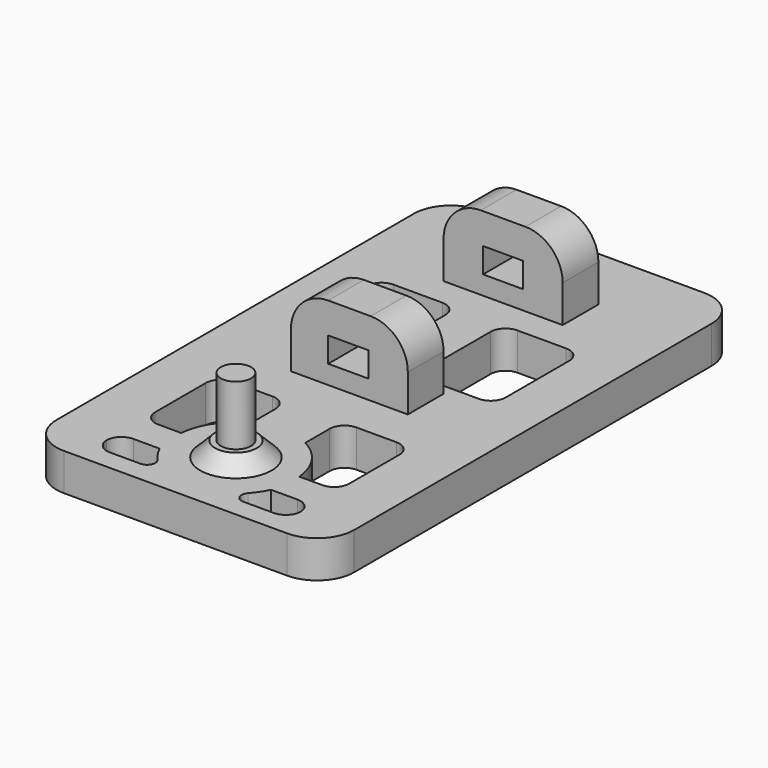
from build123d import *

# Parameters (mm, degrees)
F1_DEPTH     = 12.7
F3_DEPTH     = 25.4
F4_R         = 12.7
F5_R         = 12.7
F6_R         = 12.7
F8_DEPTH     = 104.141
F9_W         = 26.8278098665
F9_H         = 37.2433126904
F10_DEPTH    = 12.701
F11_R        = 5.08
F12_R        = 12.1917967362
F12_R_2      = 5.1797647995
F13_DEPTH    = 5.08
F14_DEPTH    = 25.4
F15_SIZE     = 5.07999
F17_DEPTH    = 25.4
F18_R        = 5.08
F19_DEPTH    = 12.701
F21_DEPTH    = 12.701
F22_T1_DEPTH = 12.7
F23_R        = 2.794


# Not quite as in the source:
# - a fillet or chamfer that OpenCascade refuses, or shapes differently, is made with other operations: its cross-section is extruded or revolved along the edge and cut away or added
# - a fillet or chamfer is up to 0.001 mm smaller than in the source, because OpenCascade refuses the exact size
# - a feature names something its author has since deleted; it is built from what else it names


with BuildPart() as f1:
    # F0 (on Top) → F1 (new body)
    with BuildSketch(Plane.XY):
        Polygon((-50.8, 88.9), (-50.8, 0), (-50.8, -88.9), (0, -88.9), (50.8, -88.9), (50.8, 0), (50.8, 88.9), (0, 88.9), align=None)
    extrude(amount=F1_DEPTH)

    # F2 (on face) → F3 (join)
    with BuildSketch(Plane.XY.offset(12.7)):
        Polygon((20.32, 66.04), (0, 66.04), (-20.32, 66.04), (-20.32, 50.8), (0, 50.8), (20.32, 50.8), align=None)
        Polygon((0, 0), (-19.5459036618, 0), (-19.5459036618, -15.24), (0, -15.24), (20.32, -15.24), (20.32, 0), align=None)
    extrude(amount=F3_DEPTH)

    # F4
    f4_edges = [f1.edges().sort_by_distance(p)[0] for p in [
        (20.32, -7.62, 38.1),
        (-19.545904, -7.62, 38.1),
    ]]
    fillet(f4_edges, radius=F4_R)

    # F5
    f5_edges = [f1.edges().sort_by_distance(p)[0] for p in [
        (20.32, 58.42, 38.1),
        (-20.32, 58.42, 38.1),
    ]]
    fillet(f5_edges, radius=F5_R)

    # F6
    f6_edges = [f1.edges().sort_by_distance(p)[0] for p in [
        (50.8, 88.9, 6.35),
        (-50.8, 88.9, 6.35),
        (50.8, -88.9, 6.35),
        (-50.8, -88.9, 6.35),
    ]]
    fillet(f6_edges, radius=F6_R)

    # F7 (on face) → F8 (cut, through all)
    with BuildSketch(Plane.XZ.offset(15.24)):
        Polygon((6.8459036618, 27.6168659329), (0, 27.6168659329), (-6.8459036618, 27.6168659329), (-6.8459036618, 19.0950892866), (0, 19.0950892866), (6.8459036618, 19.0950892866), align=None)
    extrude(amount=-F8_DEPTH, mode=Mode.SUBTRACT)

    # F9 (on face) → F10 (cut, through all)
    with BuildSketch(Plane.XY.offset(12.7)):
        with Locations((-21.1466264445, 22.2513012122)):
            Rectangle(F9_W, F9_H)
        with Locations((21.1466264445, 22.2513012122)):
            Rectangle(F9_W, F9_H)
    extrude(amount=-F10_DEPTH, mode=Mode.SUBTRACT)

    # F11
    f11_edges = [f1.edges().sort_by_distance(p)[0] for p in [
        (-34.560531, 40.872958, 6.35),
        (-7.732722, 40.872958, 6.35),
        (-7.732722, 3.629645, 6.35),
        (-34.560531, 3.629645, 6.35),
        (34.560531, 3.629645, 6.35),
        (7.732722, 3.629645, 6.35),
        (7.732722, 40.872958, 6.35),
        (34.560531, 40.872958, 6.35),
    ]]
    fillet(f11_edges, radius=F11_R)

    # F12 (on face) → F13 (join)
    with BuildSketch(Plane.XY.offset(12.7)):
        with Locations((0, -63.150562346)):
            Circle(F12_R)
        with Locations((0, -63.150562346)):
            Circle(F12_R_2, mode=Mode.SUBTRACT)
    extrude(amount=F13_DEPTH)

    # F14 (add): a face of the model
    f14_faces = [f1.faces().sort_by_distance(p)[0] for p in [
        (0, -63.150562346, 12.7),
    ]]
    extrude(f14_faces, amount=F14_DEPTH)

    # F15 (size 5.08 in the source; OpenCascade refuses exactly that, so slightly less here)
    f15_edges = [f1.edges().sort_by_distance(p)[0] for p in [
        (-12.191797, -63.150562, 17.78),
    ]]
    chamfer(f15_edges, length=F15_SIZE)

    # F16 (on face) → F17 (cut)
    with BuildSketch(Plane.XY.offset(12.7)):
        with BuildLine():
            Line((-9.2206190628, -29.6420995146), (-33.0726338262, -29.6420995146))
            Line((-33.0726338262, -29.6420995146), (-33.0726338262, -61.3056821097))
            Line((-33.0726338262, -61.3056821097), (-20.1783736468, -61.3056821097))
            ThreePointArc((-20.1783736468, -61.3056821097), (-16.7830306246, -51.7971386698), (-9.2206190628, -45.1075434685))
            Line((-9.2206190628, -45.1075434685), (-9.2206190628, -29.6420995146))
        make_face()
        with BuildLine():
            Line((33.0726338262, -29.6420995146), (9.2206190628, -29.6420995146))
            Line((9.2206190628, -29.6420995146), (9.2206190628, -45.1075434685))
            ThreePointArc((9.2206190628, -45.1075434685), (16.7830306246, -51.7971386698), (20.1783736468, -61.3056821097))
            Line((20.1783736468, -61.3056821097), (33.0726338262, -61.3056821097))
            Line((33.0726338262, -61.3056821097), (33.0726338262, -29.6420995146))
        make_face()
    extrude(amount=-F17_DEPTH, mode=Mode.SUBTRACT)

    # F18
    f18_edges = [f1.edges().sort_by_distance(p)[0] for p in [
        (-9.220619, -29.6421, 6.35),
        (-33.072634, -29.6421, 6.35),
        (-33.072634, -61.305682, 6.35),
        (33.072634, -61.305682, 6.35),
        (33.072634, -29.6421, 6.35),
        (9.220619, -29.6421, 6.35),
    ]]
    fillet(f18_edges, radius=F18_R)

    # F16 (on face) → F19 (cut, through all)
    with BuildSketch(Plane.XY.offset(12.7)):
        with BuildLine():
            Line((-9.2206190628, -29.6420995146), (-33.0726338262, -29.6420995146))
            Line((-33.0726338262, -29.6420995146), (-33.0726338262, -61.3056821097))
            Line((-33.0726338262, -61.3056821097), (-20.1783736468, -61.3056821097))
            ThreePointArc((-20.1783736468, -61.3056821097), (-16.7830306246, -51.7971386698), (-9.2206190628, -45.1075434685))
            Line((-9.2206190628, -45.1075434685), (-9.2206190628, -29.6420995146))
        make_face()
        with BuildLine():
            Line((33.0726338262, -29.6420995146), (9.2206190628, -29.6420995146))
            Line((9.2206190628, -29.6420995146), (9.2206190628, -45.1075434685))
            ThreePointArc((9.2206190628, -45.1075434685), (16.7830306246, -51.7971386698), (20.1783736468, -61.3056821097))
            Line((20.1783736468, -61.3056821097), (33.0726338262, -61.3056821097))
            Line((33.0726338262, -61.3056821097), (33.0726338262, -29.6420995146))
        make_face()
    extrude(amount=-F19_DEPTH, mode=Mode.SUBTRACT)

    # F20 (on face) → F21 (cut, through all)
    with BuildSketch(Plane.XY.offset(12.7)):
        with BuildLine():
            Line((-33.0726338262, -81.930026412), (-9.2206190628, -81.930026412))
            ThreePointArc((-9.2206190628, -81.930026412), (-14.9601496341, -77.7752677938), (-18.9837029569, -71.9430084535))
            Line((-18.9837029569, -71.9430084535), (-33.0726338262, -71.9430084535))
            Line((-33.0726338262, -71.9430084535), (-33.0726338262, -81.930026412))
        make_face()
        with BuildLine():
            ThreePointArc((18.9837029569, -71.9430084535), (14.9601496341, -77.7752677938), (9.2206190628, -81.930026412))
            Line((9.2206190628, -81.930026412), (33.0726338262, -81.930026412))
            Line((33.0726338262, -81.930026412), (33.0726338262, -71.9430084535))
            Line((33.0726338262, -71.9430084535), (18.9837029569, -71.9430084535))
        make_face()
    extrude(amount=-F21_DEPTH, mode=Mode.SUBTRACT)

    # F22: fillet of radius 5.08 on 10 edges, made by hand

    # F22_s2 → F22_t1 (join)
    with BuildSketch(Plane.XY):
        with BuildLine():
            ThreePointArc((-9.2206190628, -34.7220995146), (-10.7085166144, -31.1299970662), (-14.3006190628, -29.6420995146))
            Line((-14.3006190628, -29.6420995146), (-9.2206190628, -29.6420995146))
            Line((-9.2206190628, -29.6420995146), (-9.2206190628, -34.7220995146))
        make_face()
        with BuildLine():
            ThreePointArc((-27.9926338262, -29.6420995146), (-31.5847362746, -31.1299970662), (-33.0726338262, -34.7220995146))
            Line((-33.0726338262, -34.7220995146), (-33.0726338262, -29.6420995146))
            Line((-33.0726338262, -29.6420995146), (-27.9926338262, -29.6420995146))
        make_face()
        with BuildLine():
            ThreePointArc((-33.0726338262, -56.2256821097), (-31.5847362746, -59.8177845582), (-27.9926338262, -61.3056821097))
            Line((-27.9926338262, -61.3056821097), (-33.0726338262, -61.3056821097))
            Line((-33.0726338262, -61.3056821097), (-33.0726338262, -56.2256821097))
        make_face()
        with BuildLine():
            ThreePointArc((33.0726338262, -34.7220995146), (31.5847362746, -31.1299970662), (27.9926338262, -29.6420995146))
            Line((27.9926338262, -29.6420995146), (33.0726338262, -29.6420995146))
            Line((33.0726338262, -29.6420995146), (33.0726338262, -34.7220995146))
        make_face()
        with BuildLine():
            ThreePointArc((14.3006190628, -29.6420995146), (10.7085166144, -31.1299970662), (9.2206190628, -34.7220995146))
            Line((9.2206190628, -34.7220995146), (9.2206190628, -29.6420995146))
            Line((9.2206190628, -29.6420995146), (14.3006190628, -29.6420995146))
        make_face()
        with BuildLine():
            ThreePointArc((27.9926338262, -61.3056821097), (31.5847362746, -59.8177845582), (33.0726338262, -56.2256821097))
            Line((33.0726338262, -56.2256821097), (33.0726338262, -61.3056821097))
            Line((33.0726338262, -61.3056821097), (27.9926338262, -61.3056821097))
        make_face()
        with BuildLine():
            ThreePointArc((-33.0726338262, -76.850026412), (-31.5847362746, -80.4421288604), (-27.9926338262, -81.930026412))
            Line((-27.9926338262, -81.930026412), (-33.0726338262, -81.930026412))
            Line((-33.0726338262, -81.930026412), (-33.0726338262, -76.850026412))
        make_face()
        with BuildLine():
            ThreePointArc((-27.9926338262, -71.9430084535), (-31.5847362746, -73.4309060051), (-33.0726338262, -77.0230084535))
            Line((-33.0726338262, -77.0230084535), (-33.0726338262, -71.9430084535))
            Line((-33.0726338262, -71.9430084535), (-27.9926338262, -71.9430084535))
        make_face()
        with BuildLine():
            ThreePointArc((33.0726338262, -77.0230084535), (31.5847362746, -73.4309060051), (27.9926338262, -71.9430084535))
            Line((27.9926338262, -71.9430084535), (33.0726338262, -71.9430084535))
            Line((33.0726338262, -71.9430084535), (33.0726338262, -77.0230084535))
        make_face()
        with BuildLine():
            ThreePointArc((27.9926338262, -81.930026412), (31.5847362746, -80.4421288604), (33.0726338262, -76.850026412))
            Line((33.0726338262, -76.850026412), (33.0726338262, -81.930026412))
            Line((33.0726338262, -81.930026412), (27.9926338262, -81.930026412))
        make_face()
    extrude(amount=F22_T1_DEPTH)

    # F23
    f23_edges = [f1.edges().sort_by_distance(p)[0] for p in [
        (9.220619, -81.930026, 6.35),
        (-9.220619, -81.930026, 6.35),
    ]]
    fillet(f23_edges, radius=F23_R)


solid = f1.part
